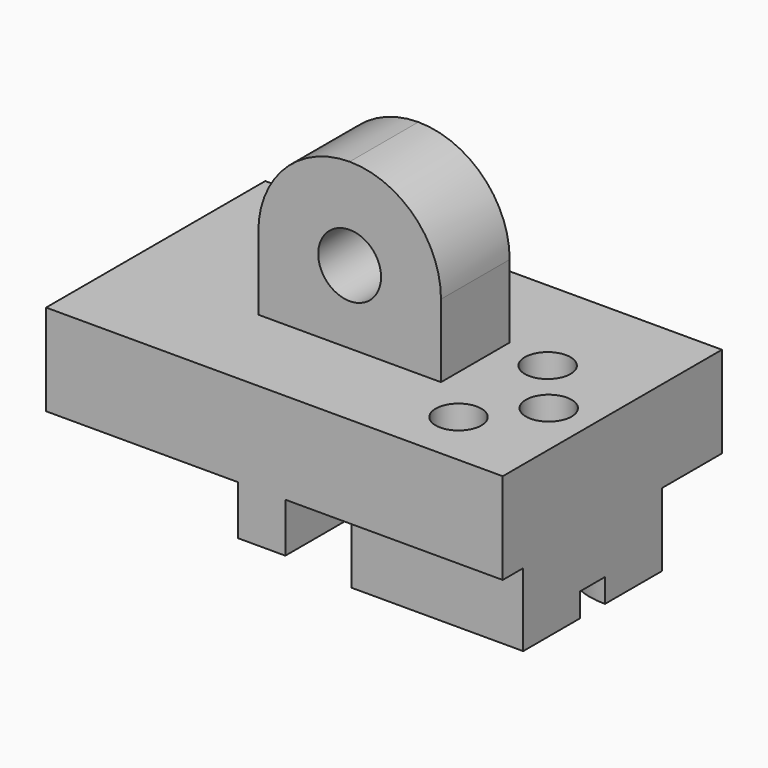
from build123d import *

# Parameters (mm, degrees)
F0_W      = 31.75
F0_H      = 6.35
F1_DEPTH  = 19.05
F2_W      = 12.7
F2_H      = 5.969
F3_DEPTH  = 11.43
F4_R      = 6.34999
F5_R      = 2.1844
F6_DEPTH  = 25.4
F7_W      = 11.938
F7_H      = 12.065
F8_DEPTH  = 5.08
F9_W      = 5.715
F9_H      = 7.747
F10_DEPTH = 1.651
F11_R     = 1.5875
F12_DEPTH = 25.4
F13_W     = 3.302
F13_H     = 19.05
F14_DEPTH = 3.429
F15_W     = 3.302
F15_H     = 6.35
F16_DEPTH = 0.635
F18_DEPTH = 1.651
F19_R     = 5.08


# Not quite as in the source:
# - a fillet or chamfer is up to 0.001 mm smaller than in the source, because OpenCascade refuses the exact size


with BuildPart() as f1:
    # F0 (on Front) → F1 (new body)
    with BuildSketch(Plane.XZ):
        Rectangle(F0_W, F0_H)
    extrude(amount=F1_DEPTH)

    # F2 (on face) → F3 (join)
    with BuildSketch(Plane.XY.offset(3.175)):
        with Locations((0, -9.525)):
            Rectangle(F2_W, F2_H)
    extrude(amount=F3_DEPTH)

    # F4 (radius 6.35 in the source; OpenCascade refuses exactly that, so slightly less here)
    f4_edges = [f1.edges().sort_by_distance(p)[0] for p in [
        (-6.35, -9.525, 14.605),
        (6.35, -9.525, 14.605),
    ]]
    fillet(f4_edges, radius=F4_R)

    # F5 (on face) → F6 (cut)
    with BuildSketch(Plane.XZ.offset(12.5095)):
        with Locations((0, 8.255)):
            Circle(F5_R)
    extrude(amount=-F6_DEPTH, mode=Mode.SUBTRACT)

    # F7 (on face) → F8 (join)
    with BuildSketch(Plane(origin=(0, 0, -3.175), x_dir=(1, 0, 0), z_dir=(0, 0, -1))):
        with Locations((9.906, 11.2395)):
            Rectangle(F7_W, F7_H)
    extrude(amount=F8_DEPTH)

    # F9 (on face) → F10 (cut)
    with BuildSketch(Plane(origin=(0, 0, -8.255), x_dir=(1, 0, 0), z_dir=(0, 0, -1))):
        with Locations((6.7945, 11.2395)):
            Rectangle(F9_W, F9_H)
    extrude(amount=-F10_DEPTH, mode=Mode.SUBTRACT)

    # F11 (on face) → F12 (cut)
    with BuildSketch(Plane(origin=(0, 0, -8.255), x_dir=(1, 0, 0), z_dir=(0, 0, -1))):
        with Locations((9.652, 15.113)):
            Circle(F11_R)
        with Locations((9.652, 7.366)):
            Circle(F11_R)
        with Locations((12.827, 11.2395)):
            Circle(F11_R)
    extrude(amount=-F12_DEPTH, mode=Mode.SUBTRACT)

    # F13 (on face) → F14 (join)
    with BuildSketch(Plane(origin=(0, 0, -3.175), x_dir=(1, 0, 0), z_dir=(0, 0, -1))):
        with Locations((-0.889, 9.525)):
            Rectangle(F13_W, F13_H)
    extrude(amount=F14_DEPTH)

    # F15 (on face) → F16 (cut)
    with BuildSketch(Plane(origin=(0, 0, -6.604), x_dir=(1, 0, 0), z_dir=(0, 0, -1))):
        with Locations((-0.889, 3.175)):
            Rectangle(F15_W, F15_H)
    extrude(amount=-F16_DEPTH, mode=Mode.SUBTRACT)

    # F17 (on face) → F18 (cut)
    with BuildSketch(Plane(origin=(0, 0, -8.255), x_dir=(1, 0, 0), z_dir=(0, 0, -1))):
        with BuildLine():
            Line((11.4142141882, 12.319), (9.652, 12.319))
            Line((9.652, 12.319), (9.652, 10.16))
            Line((9.652, 10.16), (11.4142141882, 10.16))
            ThreePointArc((11.4142141882, 10.16), (12.827, 9.4615), (14.2397858118, 10.16))
            Line((14.2397858118, 10.16), (15.875, 10.16))
            Line((15.875, 10.16), (15.875, 12.319))
            Line((15.875, 12.319), (14.2397858118, 12.319))
            ThreePointArc((14.2397858118, 12.319), (12.827, 13.0175), (11.4142141882, 12.319))
        make_face()
    extrude(amount=-F18_DEPTH, mode=Mode.SUBTRACT)

    # F19
    f19_edges = [f1.edges().sort_by_distance(p)[0] for p in [
        (11.414214, -12.319, -7.4295),
        (14.239786, -12.319, -7.4295),
        (11.414214, -10.16, -7.4295),
        (14.239786, -10.16, -7.4295),
    ]]
    fillet(f19_edges, radius=F19_R)


solid = f1.part
